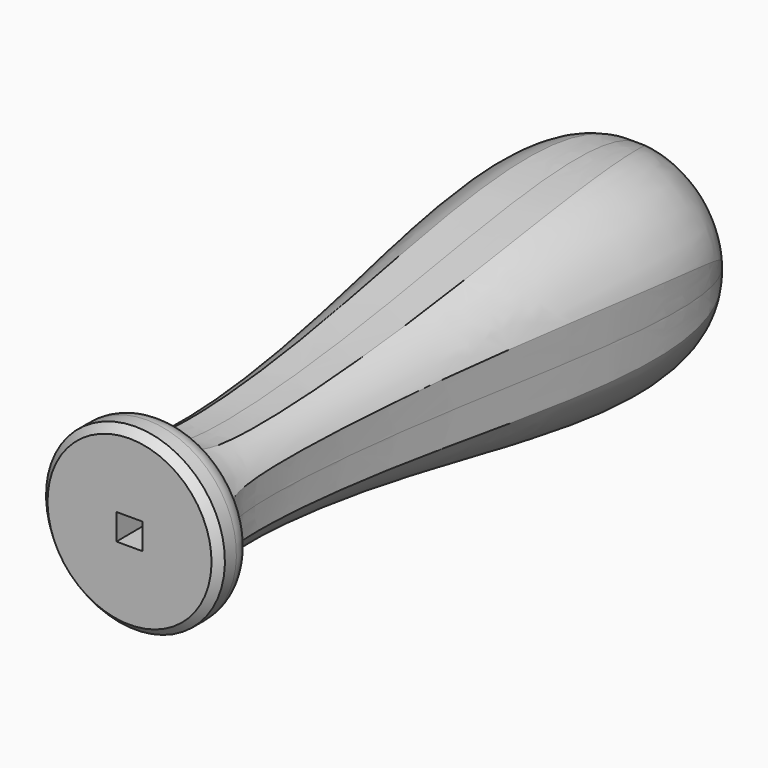
from build123d import *

# Parameters (mm, degrees)
F2_SIZE       = 1
F4_DEPTH      = 5
F4_DEPTH_BACK = 5
F5_COUNT      = 4
F7_R          = 1.5
F8_DEPTH      = 100
F8_DEPTH_BACK = 25
F9_W          = 3.5
F9_H          = 3.5
F10_DEPTH     = 25
F10_TAPER     = 2


# Not quite as in the source:
# - the dataset's text gives a spline's control points without its knots; the knots are read off the source's solid


with BuildPart() as f1:
    # F0 (on Right) → F1 (revolve)
    with BuildSketch(Plane.YZ):
        with BuildLine():
            Line((0, 12), (0, 0))
            Line((0, 0), (81.1578258872, 0))
            Line((81.1578258872, 0), (89.6560251713, 0))
            add(Edge.make_bspline(
                [(5.9228962956, 9.1504249722), (6.8900343031, 6.3685388304), (39.5618614962, 7.74400636), (85.7912643516, 19.6263415757), (89.6566016099, 4.5940827585), (89.6560251713, 0)],
                knots=[0, 0, 0, 0, 0.3442049299, 0.770390417, 1, 1, 1, 1], degree=3))
            ThreePointArc((5.9228962956, 9.1504249722), (4.9941231012, 11.1738531363), (2.9266699477, 12))
            Line((2.9266699477, 12), (0, 12))
        make_face()
    revolve(axis=Axis((0, 40.5789129436, 0), (0, -1, 0)))

    # F2
    f2_edges = [f1.edges().sort_by_distance(p)[0] for p in [
        (0, 0, -12),
    ]]
    chamfer(f2_edges, length=F2_SIZE)


with BuildPart() as f4:
    # F3 (on Right) → F4 (new body, two sides)
    with BuildSketch(Plane.YZ) as f4_sk:
        with BuildLine():
            Line((9.9051892757, 31.0736633837), (5.8965189382, 9.1559858993))
            add(Edge.make_bspline(
                [(5.8965189382, 9.1559858993), (5.9472195677, 9.0115264008), (6.0787007332, 8.737855916), (6.4264167356, 8.2752529498), (6.9540357429, 7.8492817721), (7.6695442866, 7.4849318101), (8.477817305, 7.2057885171), (9.3889273865, 6.9862523042), (10.7476798966, 6.7569867165), (12.7180994024, 6.573641292), (15.4916643071, 6.4956271004), (18.6289754692, 6.5476748187), (22.078511792, 6.7198568853), (27.0212738393, 7.0977311992), (32.3663475985, 7.6806858139), (37.8866306932, 8.4350672988), (42.0526870012, 9.0778266944), (46.2117571502, 9.7683310663), (51.7119278945, 10.714634681), (58.4302704603, 11.8739992087), (66.0089075261, 12.9994054756), (72.8627638727, 13.633285281), (77.7556936417, 13.5687704983), (81.0348580655, 13.0706857657), (82.7880556534, 12.5628486358), (83.9981341745, 12.0377737343), (85.0789008782, 11.432460952), (86.1265707678, 10.6022255642), (86.8008379577, 9.8405494507), (87.0694741607, 9.4896582887)],
                knots=[0, 0, 0, 0, 0.0078125, 0.015625, 0.03125, 0.046875, 0.0625, 0.078125, 0.09375, 0.125, 0.15625, 0.1875, 0.21875, 0.25, 0.3125, 0.34375, 0.375, 0.40625, 0.4375, 0.5, 0.5625, 0.625, 0.6875, 0.71875, 0.75, 0.765625, 0.78125, 0.8125, 0.8365570463, 0.8365570463, 0.8365570463, 0.8365570463], degree=3))
            Line((87.0694741607, 9.4896582887), (93.1284055114, 31.0736633837))
            Line((93.1284055114, 31.0736633837), (9.9051892757, 31.0736633837))
        make_face()
    extrude(amount=F4_DEPTH)
    extrude(f4_sk.sketch, amount=-F4_DEPTH_BACK)


with BuildPart() as f5_1:
    # F5: instance of F4
    add(f4.part.rotate(Axis((0, 0, 0), (0, -1, 0)), 1 * 360 / F5_COUNT))


with BuildPart() as f5_2:
    # F5: instance of F4
    add(f4.part.rotate(Axis((0, 0, 0), (0, -1, 0)), 2 * 360 / F5_COUNT))


with BuildPart() as f5_3:
    # F5: instance of F4
    add(f4.part.rotate(Axis((0, 0, 0), (0, -1, 0)), 3 * 360 / F5_COUNT))


with BuildPart() as f1_1:
    add(f1.part)

    # F6: cut F4, F5_1, F5_2, F5_3
    add(f4.part, mode=Mode.SUBTRACT)
    add(f5_1.part, mode=Mode.SUBTRACT)
    add(f5_2.part, mode=Mode.SUBTRACT)
    add(f5_3.part, mode=Mode.SUBTRACT)

    # F7 (on Front) → F8 (cut, two sides)
    with BuildSketch(Plane.XZ) as f8_sk:
        Circle(F7_R)
    extrude(amount=-F8_DEPTH, mode=Mode.SUBTRACT)
    extrude(f8_sk.sketch, amount=F8_DEPTH_BACK, mode=Mode.SUBTRACT)

    # F9 (on Front) → F10 (cut)
    with BuildSketch(Plane.XZ):
        Rectangle(F9_W, F9_H)
    extrude(amount=-F10_DEPTH, taper=F10_TAPER, mode=Mode.SUBTRACT)


solid = f1_1.part
